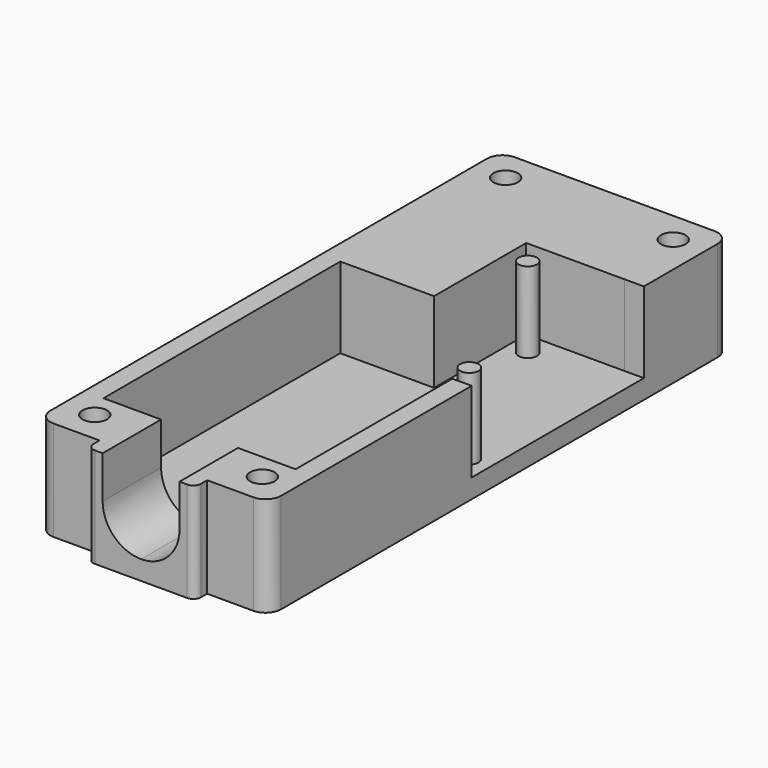
from build123d import *

# Parameters (mm, degrees)
F0_W      = 30
F0_H      = 55
F1_DEPTH  = 13
F2_T      = -2.5
F3_W      = 2.5
F3_H      = 28
F4_DEPTH  = 10.5
F6_W      = 30
F6_H      = 13
F7_DEPTH  = 10
F9_R      = 2
F10_DEPTH = 10
F11_W     = 10
F11_H     = 7.5
F12_DEPTH = 10.5
F11_R     = 1.6
F13_DEPTH = 13.5
F5_W      = 12.8000527501
F5_H      = 1.513499856
F5_R      = 1.2
F14_DEPTH = 13
F16_R     = 2
F18_DEPTH = 2
F19_R     = 1
F20_R     = 4.99999


# Not quite as in the source:
# - a fillet or chamfer is up to 0.001 mm smaller than in the source, because OpenCascade refuses the exact size
# - a feature of the source that left no trace in its solid (it failed there, or was rolled back) is left out
# - a pattern or mirror of a feature is missing from the dataset's text; its kind, count and spacing are read off the source's solid
# - a feature names something its author has since deleted; it is built from what else it names


with BuildPart() as f1:
    # F0 (on Top) → F1 (new body)
    with BuildSketch(Plane.XY):
        with Locations((2.1054805815, 0.7215001613)):
            Rectangle(F0_W, F0_H)
    extrude(amount=F1_DEPTH)

    # F2
    f2_openings = [f1.faces().sort_by_distance(p)[0] for p in [
        (2.105481, 0.7215, 13),
    ]]
    offset(amount=F2_T, openings=f2_openings)

    # F3 (on face) → F4 (cut)
    with BuildSketch(Plane.XY.offset(13)):
        with Locations((15.8554805815, 10.2215001613)):
            Rectangle(F3_W, F3_H)
    extrude(amount=-F4_DEPTH, mode=Mode.SUBTRACT)

    # F6 (on face) → F7 (join)
    with BuildSketch(Plane(origin=(0, 28.2215001613, 0), x_dir=(-1, 0, 0), z_dir=(0, 1, 0))):
        with Locations((-2.1054805815, 6.5)):
            Rectangle(F6_W, F6_H)
    extrude(amount=F7_DEPTH)

    # F9
    f9_edges = [f1.edges().sort_by_distance(p)[0] for p in [
        (17.105481, 38.2215, 6.5),
        (-12.894519, 38.2215, 6.5),
    ]]
    fillet(f9_edges, radius=F9_R)

    # F10 (add): a face of the model
    f10_faces = [f1.faces().sort_by_distance(p)[0] for p in [
        (2.1054805815, -26.7784998387, 6.5),
    ]]
    extrude(f10_faces, amount=F10_DEPTH)

    # F11 (on face) → F12 (cut)
    with BuildSketch(Plane.XY.offset(13)):
        Polygon((14.6054805815, -24.2784998387), (-10.3945194185, -24.2784998387), (-10.3945194185, -29.2784998387), (-2.8945194185, -29.2784998387), (7.1054805815, -29.2784998387), (14.6054805815, -29.2784998387), align=None)
        with Locations((2.1054805815, -33.0284998387)):
            Rectangle(F11_W, F11_H)
    extrude(amount=-F12_DEPTH, mode=Mode.SUBTRACT)

    # F11 (on face) → F13 (cut)
    with BuildSketch(Plane.XY.offset(13)):
        with Locations((13.0054805815, -32.6784998387)):
            Circle(F11_R)
        with Locations((-8.7945194185, -32.6784998387)):
            Circle(F11_R)
    f13 = extrude(amount=-F13_DEPTH, mode=Mode.SUBTRACT)

    # F13_copies: F13 across plane
    add(f13.mirror(Plane.ZX.offset(0.7215)), mode=Mode.SUBTRACT)

    # F5 (on face) → F14 (join)
    with BuildSketch(Plane.XY):
        Polygon((1.8054805815, 25.7350058258), (-10.3945194185, 25.7350058258), (-10.3945194185, 9.2350058258), (1.8054805815, 9.2350058258), (1.8054805815, 24.2215059698), align=None)
        with Locations((8.2055069566, 24.9782558978)):
            Rectangle(F5_W, F5_H)
        with Locations((4.4054805815, 21.2215001613)):
            Circle(F5_R)
        with Locations((14.4054805815, -0.7784998387)):
            Circle(F5_R)
    extrude(amount=F14_DEPTH)

    # F16
    f16_edges = [f1.edges().sort_by_distance(p)[0] for p in [
        (17.105481, -36.7785, 6.5),
        (-12.894519, -36.7785, 6.5),
    ]]
    fillet(f16_edges, radius=F16_R)

    # F17 (on face) → F18 (join)
    with BuildSketch(Plane.XZ.offset(36.7784998387)):
        Polygon((-2.8945194185, 13), (-4.8945194185, 13), (-4.8945194185, 0), (9.1054805815, 0), (9.1054805815, 13), (7.1054805815, 13), (7.1054805815, 2.5), (-2.8945194185, 2.5), align=None)
    extrude(amount=F18_DEPTH)

    # F19
    f19_edges = [f1.edges().sort_by_distance(p)[0] for p in [
        (-4.894519, -38.7785, 6.5),
        (9.105481, -38.7785, 6.5),
    ]]
    fillet(f19_edges, radius=F19_R)

    # F20 (radius 5 in the source; OpenCascade refuses exactly that, so slightly less here)
    f20_edges = [f1.edges().sort_by_distance(p)[0] for p in [
        (-2.894519, -34.0285, 2.5),
        (7.105481, -34.0285, 2.5),
    ]]
    fillet(f20_edges, radius=F20_R)


solid = f1.part
